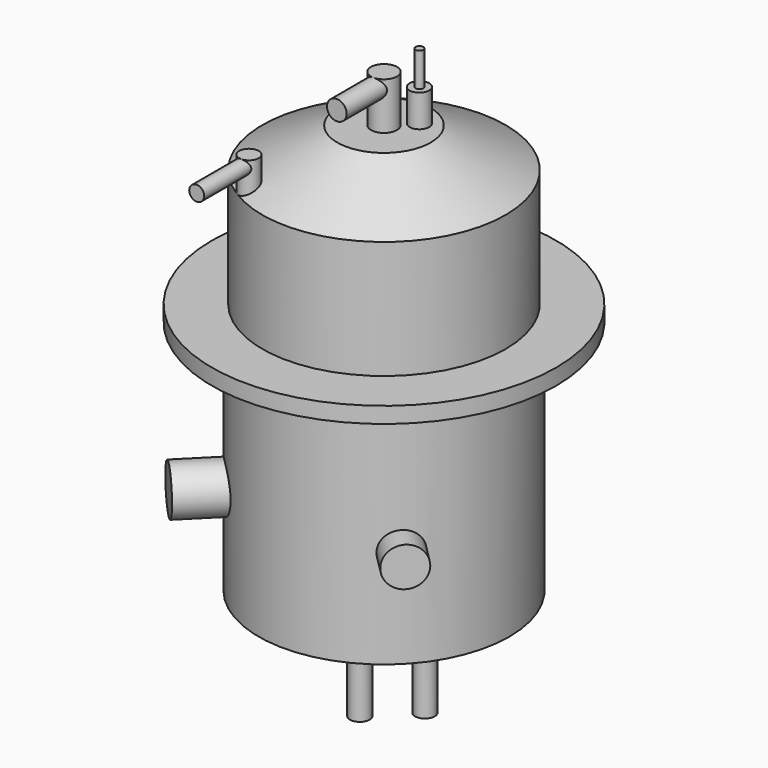
from build123d import *

# Parameters (mm, degrees)
F0_R      = 40.48125
F1_DEPTH  = 76.2
F2_R      = 55.5625
F3_DEPTH  = 5.159375
F4_R      = 39.290625
F5_DEPTH  = 38.1
F10_R     = 7.62
F11_DEPTH = 54.61
F12_R     = 6.35
F13_DEPTH = 48.514
F14_R     = 3.175
F15_DEPTH = 12.7
F16_R     = 3.175
F17_DEPTH = 25.4
F18_R     = 4.191
F19_DEPTH = 15.24
F20_R     = 3.175
F21_DEPTH = 19.05
F22_R     = 3.175
F23_DEPTH = 10.414
F24_R     = 1.27
F25_DEPTH = 10.922
F26_R     = 3.175
F27_DEPTH = 48.768
F30_R     = 2.413
F31_DEPTH = 21.082


with BuildPart() as f1:
    # F0 (on Top) → F1 (new body)
    with BuildSketch(Plane.XY):
        Circle(F0_R)
    extrude(amount=-F1_DEPTH)

    # F2 (on face) → F3 (join)
    with BuildSketch(Plane.XY):
        Circle(F2_R)
    extrude(amount=F3_DEPTH)

    # F4 (on face) → F5 (join)
    with BuildSketch(Plane.XY.offset(5.159375)):
        Circle(F4_R)
    extrude(amount=F5_DEPTH)

    # F6 (on Front) → F7 (revolve)
    with BuildSketch(Plane.XZ):
        Polygon((15.08125, 55.959375), (0, 55.959375), (0, 43.259375), (39.290625, 43.259375), align=None)
    revolve(axis=Axis((0, 0, 49.609375), (0, 0, -1)))

    # F10 (on face) → F11 (join)
    with BuildSketch(Plane(origin=(0, 0, 0), x_dir=(0.7071067812, -0.7071067812, 0), z_dir=(-0.7071067812, -0.7071067812, 0))):
        with Locations((0, -44.45)):
            Circle(F10_R)
    extrude(amount=F11_DEPTH)

    # F12 (on face) → F13 (join)
    with BuildSketch(Plane(origin=(0, 0, 0), x_dir=(0.7071067812, 0.7071067812, 0), z_dir=(0.7071067812, -0.7071067812, 0))):
        with Locations((0, -44.45)):
            Circle(F12_R)
    extrude(amount=F13_DEPTH)

    # F14 (on face) → F15 (join)
    with BuildSketch(Plane(origin=(0, 0, -76.2), x_dir=(1, 0, 0), z_dir=(0, 0, -1))):
        Circle(F14_R)
    extrude(amount=F15_DEPTH)

    # F16 (on face) → F17 (join)
    with BuildSketch(Plane(origin=(0, 0, -76.2), x_dir=(1, 0, 0), z_dir=(0, 0, -1))):
        with Locations((7.6332177029, 19.3075506603)):
            Circle(F16_R)
        with Locations((19.3075506603, 7.6332177029)):
            Circle(F16_R)
    extrude(amount=F17_DEPTH)

    # F18 (on face) → F19 (join)
    with BuildSketch(Plane.XY.offset(55.959375)):
        Circle(F18_R)
    extrude(amount=F19_DEPTH)

    # F20 (on Front) → F21 (join)
    with BuildSketch(Plane.XZ):
        with Locations((0, 68.024375)):
            Circle(F20_R)
    extrude(amount=F21_DEPTH)

    # F22 (on face) → F23 (join)
    with BuildSketch(Plane.XY.offset(55.959375)):
        with Locations((6.35, 6.35)):
            Circle(F22_R)
    extrude(amount=F23_DEPTH)

    # F24 (on face) → F25 (join)
    with BuildSketch(Plane.XY.offset(66.373375)):
        with Locations((6.35, 6.35)):
            Circle(F24_R)
    extrude(amount=F25_DEPTH)

    # F26 (on face) → F27 (join)
    with BuildSketch(Plane.XY.offset(5.159375)):
        with Locations((-19.05, -30.6828269418)):
            Circle(F26_R)
    extrude(amount=F27_DEPTH)

    # F30 (on plane+point) → F31 (join)
    with BuildSketch(Plane.XZ.offset(30.6828269418)):
        with Locations((-19.05, 51.514375)):
            Circle(F30_R)
    extrude(amount=F31_DEPTH)


solid = f1.part
